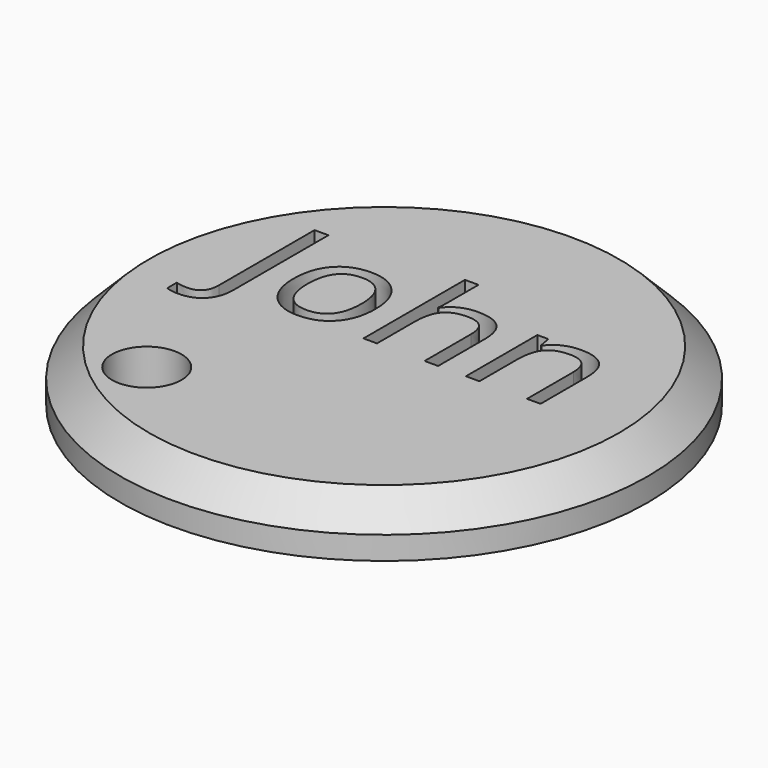
from build123d import *

# Parameters (mm, degrees)
F0_R         = 45.7999897165
F1_DEPTH     = 9
F2_SIZE      = 5
F3_TEXT_SIZE = 28.9601273835
F5_DEPTH     = 6
F4_R         = 6.0347899186
F6_DEPTH     = 11


# Not quite as in the source:
# - Text() gives the source's letters only with a copy of the font that has no kerning and outlines rounded to 1/6400 em; it was checked with that copy


with BuildPart() as f1:
    # F0 (on Top) → F1 (new body)
    with BuildSketch(Plane.XY):
        Circle(F0_R)
    extrude(amount=F1_DEPTH)

    # F2
    f2_edges = [f1.edges().sort_by_distance(p)[0] for p in [
        (-45.79999, 0, 9),
    ]]
    chamfer(f2_edges, length=F2_SIZE)

    # F3 (on face) → F5 (cut)
    with BuildSketch(Plane.XY.offset(9)):
        with Locations((-31.2927751438, 0)):
            Text('John', F3_TEXT_SIZE, font='Open Sans', text_align=(TextAlign.LEFT, TextAlign.BOTTOM))
    extrude(amount=-F5_DEPTH, mode=Mode.SUBTRACT)

    # F4 (on face) → F6 (cut)
    with BuildSketch(Plane.XY.offset(9)):
        with Locations((-21.2392248213, -24.9245688319)):
            Circle(F4_R)
    extrude(amount=-F6_DEPTH, mode=Mode.SUBTRACT)


solid = f1.part
